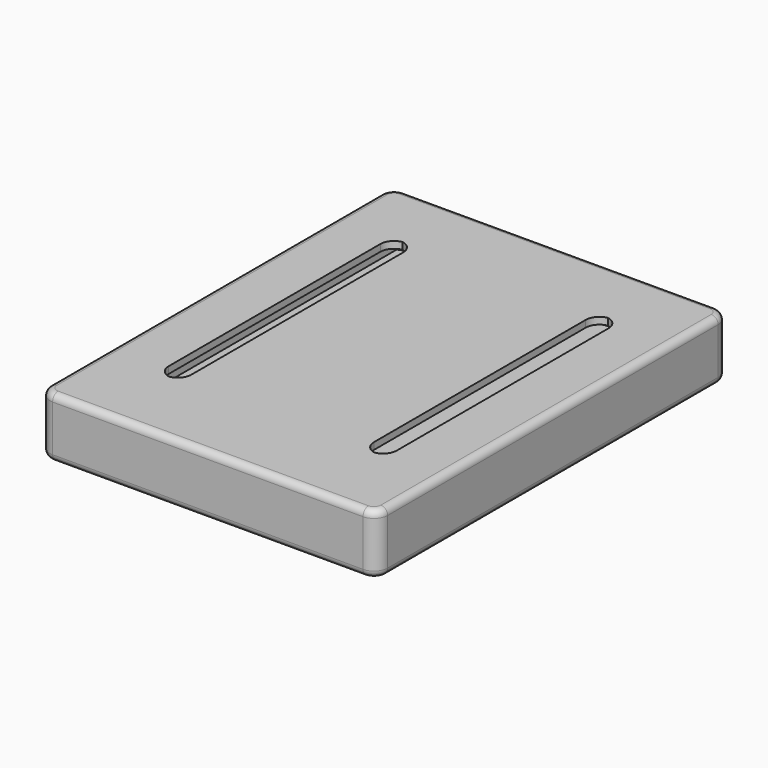
from build123d import *

# Parameters (mm, degrees)
F0_W        = 74
F0_H        = 13.15
F0_W_2      = 71
F0_H_2      = 10.15
F1_DEPTH    = 96.5
F2_DEPTH    = 95
F3_W        = 5
F3_H        = 64
F4_DEPTH    = 3
F5_T1_DEPTH = 28.15
F6_T1_DEPTH = 1.5
F7_R        = 1.49999


# Not quite as in the source:
# - a fillet or chamfer that OpenCascade refuses, or shapes differently, is made with other operations: its cross-section is extruded or revolved along the edge and cut away or added
# - a fillet or chamfer is up to 0.001 mm smaller than in the source, because OpenCascade refuses the exact size


with BuildPart() as f1:
    # F0 (on Front) → F1 (new body)
    with BuildSketch(Plane.XZ):
        Rectangle(F0_W, F0_H)
        Rectangle(F0_W_2, F0_H_2, mode=Mode.SUBTRACT)
        Rectangle(F0_W_2, F0_H_2)
    extrude(amount=F1_DEPTH)

    # F0 (on Front) → F2 (cut)
    with BuildSketch(Plane.XZ):
        Rectangle(F0_W_2, F0_H_2)
    extrude(amount=F2_DEPTH, mode=Mode.SUBTRACT)

    # F3 (on face) → F4 (cut)
    with BuildSketch(Plane.XY.offset(6.575)):
        with Locations((22.5, -47)):
            Rectangle(F3_W, F3_H)
        with Locations((-22.5, -47)):
            Rectangle(F3_W, F3_H)
    extrude(amount=-F4_DEPTH, mode=Mode.SUBTRACT)

    # F5: fillet of radius 3 on 4 edges, made by hand

    # F5_s2 → F5_t1 (cut)
    with BuildSketch(Plane.XY.offset(-14.075)):
        with BuildLine():
            ThreePointArc((37, -93.5), (36.1213203436, -95.6213203436), (34, -96.5))
            Line((34, -96.5), (37, -96.5))
            Line((37, -96.5), (37, -93.5))
        make_face()
        with BuildLine():
            ThreePointArc((-34, 0), (-36.1213203436, -0.8786796564), (-37, -3))
            Line((-37, -3), (-37, 0))
            Line((-37, 0), (-34, 0))
        make_face()
        with BuildLine():
            ThreePointArc((37, -3), (36.1213203436, -0.8786796564), (34, 0))
            Line((34, 0), (37, 0))
            Line((37, 0), (37, -3))
        make_face()
        with BuildLine():
            ThreePointArc((-34, -96.5), (-36.1213203436, -95.6213203436), (-37, -93.5))
            Line((-37, -93.5), (-37, -96.5))
            Line((-37, -96.5), (-34, -96.5))
        make_face()
    extrude(amount=F5_T1_DEPTH, mode=Mode.SUBTRACT)

    # F6: fillet of radius 3 on 8 edges, made by hand

    # F6_s2 → F6_t1 (join)
    with BuildSketch(Plane.XY.offset(5.075)):
        with BuildLine():
            ThreePointArc((25, -76), (24.1213203436, -78.1213203436), (22, -79))
            Line((22, -79), (25, -79))
            Line((25, -79), (25, -76))
        make_face()
        with BuildLine():
            ThreePointArc((23, -15), (20.8786796564, -15.8786796564), (20, -18))
            Line((20, -18), (20, -15))
            Line((20, -15), (23, -15))
        make_face()
        with BuildLine():
            ThreePointArc((25, -18), (24.1213203436, -15.8786796564), (22, -15))
            Line((22, -15), (25, -15))
            Line((25, -15), (25, -18))
        make_face()
        with BuildLine():
            ThreePointArc((23, -79), (20.8786796564, -78.1213203436), (20, -76))
            Line((20, -76), (20, -79))
            Line((20, -79), (23, -79))
        make_face()
        with BuildLine():
            ThreePointArc((-23, -79), (-20.8786796564, -78.1213203436), (-20, -76))
            Line((-20, -76), (-20, -79))
            Line((-20, -79), (-23, -79))
        make_face()
        with BuildLine():
            ThreePointArc((-25, -18), (-24.1213203436, -15.8786796564), (-22, -15))
            Line((-22, -15), (-25, -15))
            Line((-25, -15), (-25, -18))
        make_face()
        with BuildLine():
            ThreePointArc((-22, -79), (-24.1213203436, -78.1213203436), (-25, -76))
            Line((-25, -76), (-25, -79))
            Line((-25, -79), (-22, -79))
        make_face()
        with BuildLine():
            ThreePointArc((-20, -18), (-20.8786796564, -15.8786796564), (-23, -15))
            Line((-23, -15), (-20, -15))
            Line((-20, -15), (-20, -18))
        make_face()
    extrude(amount=F6_T1_DEPTH)

    # F7 (radius 1.5 in the source; OpenCascade refuses exactly that, so slightly less here)
    f7_edges = [f1.edges().sort_by_distance(p)[0] for p in [
        (0, -96.5, 6.575),
        (37, -48.25, 6.575),
        (-37, -48.25, 6.575),
        (0, -96.5, -6.575),
        (37, -48.25, -6.575),
        (-37, -48.25, -6.575),
    ]]
    fillet(f7_edges, radius=F7_R)


solid = f1.part
